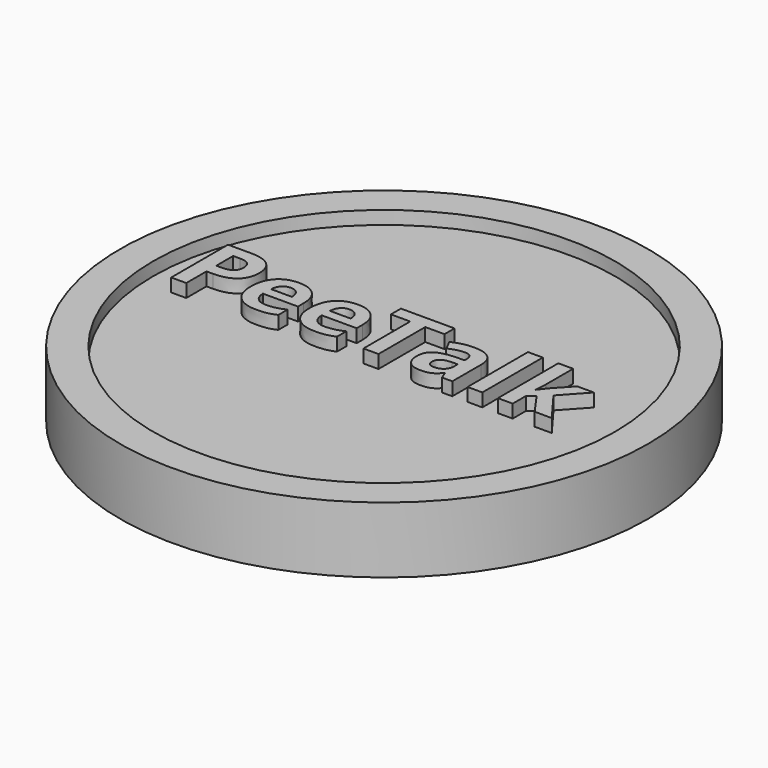
from build123d import *

# Parameters (mm, degrees)
F0_R         = 20
F1_DEPTH     = 5
F2_R         = 17.5
F3_DEPTH     = 1
F4_TEXT_SIZE = 7.5323656336
F5_DEPTH     = 1


# Not quite as in the source:
# - Text() gives the source's letters only with a copy of the font that has no kerning and outlines rounded to 1/6400 em; it was checked with that copy


with BuildPart() as f1:
    # F0 (on Top) → F1 (new body)
    with BuildSketch(Plane.XY):
        Circle(F0_R)
    extrude(amount=F1_DEPTH)

    # F2 (on face) → F3 (cut)
    with BuildSketch(Plane.XY.offset(5)):
        Circle(F2_R)
    extrude(amount=-F3_DEPTH, mode=Mode.SUBTRACT)


with BuildPart() as f5:
    # F4 (on face) → F5 (new body)
    with BuildSketch(Plane.XY.offset(5)):
        with Locations((-14.8352806951, -2.4632915582)):
            Text('PeeTalk', F4_TEXT_SIZE, font='Open Sans', font_style=FontStyle.BOLD, text_align=(TextAlign.LEFT, TextAlign.BOTTOM))
    extrude(amount=F5_DEPTH)


solid = Compound([f1.part, f5.part])
